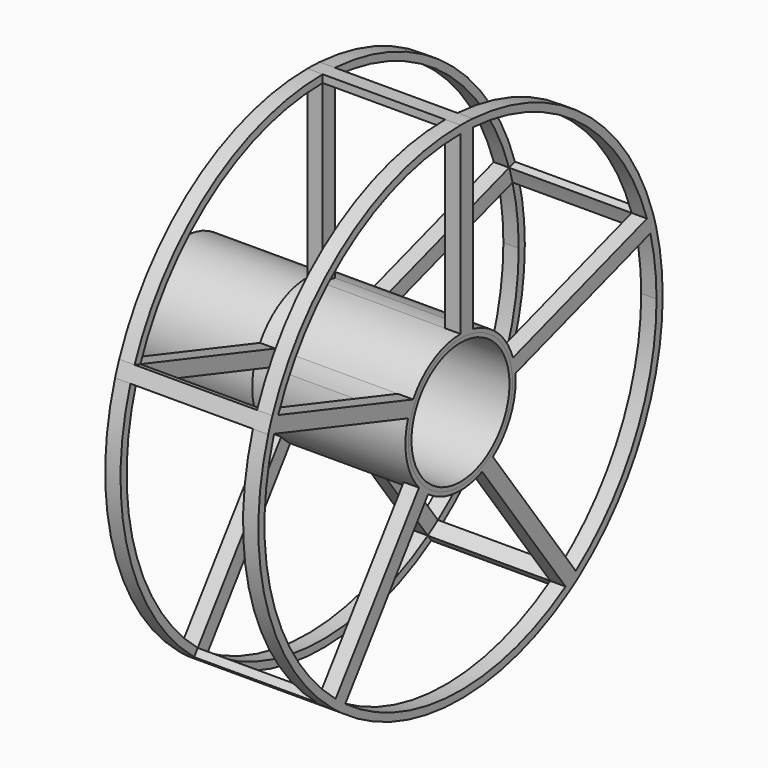
from build123d import *

# Parameters (mm, degrees)
F0_R          = 13.49375
F1_DEPTH      = 3.175
F2_DEPTH      = 28.575
F3_START      = 28.575
F3_DEPTH      = 3.175
F0_R_2        = 12.7
F4_DEPTH      = 31.75
F4_DEPTH_BACK = 25.4
F5_DEPTH      = 31.75


with BuildPart() as f1:
    # F0 (on Right) → F1 (new body)
    with BuildSketch(Plane.YZ):
        with BuildLine():
            ThreePointArc((3.175, 50.700684), (31.129836, 40.144406), (48.313671, 15.698063))
            Line((48.313671, 15.698063), (49.823473, 16.188628))
            ThreePointArc((49.823473, 16.188628), (32.063351, 41.429358), (3.175, 52.291199))
            Line((3.175, 52.291199), (3.175, 50.700684))
        make_face()
        with BuildLine():
            Line((28.167367, -44.170687), (27.232485, -42.883933))
            ThreePointArc((27.232485, -42.883933), (-1.588276, -50.775165), (-29.859491, -41.098063))
            Line((-29.859491, -41.098063), (-30.7926, -42.382378))
            ThreePointArc((-30.7926, -42.382378), (-1.58823, -52.363419), (28.167367, -44.170687))
        make_face()
        with BuildLine():
            ThreePointArc((0, 50.8), (1.588276, 50.775165), (3.175, 50.700684))
            Line((3.175, 50.700684), (3.175, 52.291199))
            ThreePointArc((3.175, 52.291199), (1.58823, 52.363419), (0, 52.3875))
            Line((0, 52.3875), (0, 50.8))
        make_face()
        with BuildLine():
            ThreePointArc((48.313671, 15.698063), (48.780856, 14.179848), (49.200345, 12.647769))
            Line((49.200345, 12.647769), (50.713015, 13.139265))
            ThreePointArc((50.713015, 13.139265), (50.291361, 14.67069), (49.823473, 16.188628))
            Line((49.823473, 16.188628), (48.313671, 15.698063))
        make_face()
        with BuildLine():
            ThreePointArc((49.200345, 12.647769), (50.3985, 6.374264), (50.8, 0))
            ThreePointArc((50.8, 0), (45.263131, -23.062717), (29.859491, -41.098063))
            Line((29.859491, -41.098063), (30.7926, -42.382378))
            ThreePointArc((30.7926, -42.382378), (46.677604, -23.783427), (52.3875, 0))
            ThreePointArc((52.3875, 0), (51.967193, 6.622767), (50.713015, 13.139265))
            Line((50.713015, 13.139265), (49.200345, 12.647769))
        make_face()
        with BuildLine():
            ThreePointArc((-47.238087, 18.686977), (-28.55995, 42.011537), (0, 50.8))
            Line((0, 50.8), (0, 52.3875))
            ThreePointArc((0, 52.3875), (-29.493541, 43.296434), (-48.750757, 19.178474))
            Line((-48.750757, 19.178474), (-47.238087, 18.686977))
        make_face()
        with BuildLine():
            Line((-33.304625, -40.438251), (-32.369743, -39.151497))
            ThreePointArc((-32.369743, -39.151497), (-48.780856, -14.179848), (-48.313671, 15.698063))
            Line((-48.313671, 15.698063), (-49.823473, 16.188628))
            ThreePointArc((-49.823473, 16.188628), (-50.291361, -14.67069), (-33.304625, -40.438251))
        make_face()
        with BuildLine():
            ThreePointArc((-48.313671, 15.698063), (-47.799247, 17.20093), (-47.238087, 18.686977))
            Line((-47.238087, 18.686977), (-48.750757, 19.178474))
            ThreePointArc((-48.750757, 19.178474), (-49.309781, 17.691683), (-49.823473, 16.188628))
            Line((-49.823473, 16.188628), (-48.313671, 15.698063))
        make_face()
        with BuildLine():
            Line((30.7926, -42.382378), (29.859491, -41.098063))
            ThreePointArc((29.859491, -41.098063), (28.55995, -42.011537), (27.232485, -42.883933))
            Line((27.232485, -42.883933), (28.167367, -44.170687))
            ThreePointArc((28.167367, -44.170687), (29.493541, -43.296434), (30.7926, -42.382378))
        make_face()
        with BuildLine():
            ThreePointArc((-32.369743, -39.151497), (-31.129836, -40.144406), (-29.859491, -41.098063))
            Line((-29.859491, -41.098063), (-8.397982, -11.55883))
            ThreePointArc((-8.397982, -11.55883), (-9.63774, -10.547352), (-10.756628, -9.403596))
            Line((-10.756628, -9.403596), (-32.369743, -39.151497))
        make_face()
        with BuildLine():
            Line((14.22959, 1.285081), (49.200345, 12.647769))
            ThreePointArc((49.200345, 12.647769), (48.780856, 14.179848), (48.313671, 15.698063))
            Line((48.313671, 15.698063), (13.58822, 4.41508))
            ThreePointArc((13.58822, 4.41508), (13.996673, 2.868065), (14.22959, 1.285081))
        make_face()
        with BuildLine():
            ThreePointArc((27.232485, -42.883933), (28.55995, -42.011537), (29.859491, -41.098063))
            Line((29.859491, -41.098063), (8.397982, -11.55883))
            ThreePointArc((8.397982, -11.55883), (7.052902, -12.425346), (5.61937, -13.136032))
            Line((5.61937, -13.136032), (27.232485, -42.883933))
        make_face()
        with BuildLine():
            Line((3.175, 13.930256), (3.175, 50.700684))
            ThreePointArc((3.175, 50.700684), (1.588276, 50.775165), (0, 50.8))
            Line((0, 50.8), (0, 14.2875))
            ThreePointArc((0, 14.2875), (1.597517, 14.197908), (3.175, 13.930256))
        make_face()
        with BuildLine():
            Line((-30.7926, -42.382378), (-29.859491, -41.098063))
            ThreePointArc((-29.859491, -41.098063), (-31.129836, -40.144406), (-32.369743, -39.151497))
            Line((-32.369743, -39.151497), (-33.304625, -40.438251))
            ThreePointArc((-33.304625, -40.438251), (-32.063351, -41.429358), (-30.7926, -42.382378))
        make_face()
        with BuildLine():
            ThreePointArc((14.2875, 0), (14.273015, 0.643193), (14.22959, 1.285081))
            ThreePointArc((14.22959, 1.285081), (13.996673, 2.868065), (13.58822, 4.41508))
            ThreePointArc((13.58822, 4.41508), (9.63774, 10.547352), (3.175, 13.930256))
            ThreePointArc((3.175, 13.930256), (1.597517, 14.197908), (0, 14.2875))
            ThreePointArc((0, 14.2875), (-7.052902, 12.425346), (-12.267332, 7.32429))
            ThreePointArc((-12.267332, 7.32429), (-13.009353, 5.906724), (-13.58822, 4.41508))
            ThreePointArc((-13.58822, 4.41508), (-13.996673, -2.868065), (-10.756628, -9.403596))
            ThreePointArc((-10.756628, -9.403596), (-9.63774, -10.547352), (-8.397982, -11.55883))
            ThreePointArc((-8.397982, -11.55883), (-1.597517, -14.197908), (5.61937, -13.136032))
            ThreePointArc((5.61937, -13.136032), (7.052902, -12.425346), (8.397982, -11.55883))
            ThreePointArc((8.397982, -11.55883), (12.730256, -6.486389), (14.2875, 0))
        make_face()
        Circle(F0_R, mode=Mode.SUBTRACT)
        with BuildLine():
            Line((-12.267332, 7.32429), (-47.238087, 18.686977))
            ThreePointArc((-47.238087, 18.686977), (-47.799247, 17.20093), (-48.313671, 15.698063))
            Line((-48.313671, 15.698063), (-13.58822, 4.41508))
            ThreePointArc((-13.58822, 4.41508), (-13.009353, 5.906724), (-12.267332, 7.32429))
        make_face()
    extrude(amount=F1_DEPTH)

    # F0 (on Right) → F2 (join)
    with BuildSketch(Plane.YZ):
        with BuildLine():
            ThreePointArc((48.313671, 15.698063), (48.780856, 14.179848), (49.200345, 12.647769))
            Line((49.200345, 12.647769), (50.713015, 13.139265))
            ThreePointArc((50.713015, 13.139265), (50.291361, 14.67069), (49.823473, 16.188628))
            Line((49.823473, 16.188628), (48.313671, 15.698063))
        make_face()
        with BuildLine():
            Line((-30.7926, -42.382378), (-29.859491, -41.098063))
            ThreePointArc((-29.859491, -41.098063), (-31.129836, -40.144406), (-32.369743, -39.151497))
            Line((-32.369743, -39.151497), (-33.304625, -40.438251))
            ThreePointArc((-33.304625, -40.438251), (-32.063351, -41.429358), (-30.7926, -42.382378))
        make_face()
        with BuildLine():
            ThreePointArc((0, 50.8), (1.588276, 50.775165), (3.175, 50.700684))
            Line((3.175, 50.700684), (3.175, 52.291199))
            ThreePointArc((3.175, 52.291199), (1.58823, 52.363419), (0, 52.3875))
            Line((0, 52.3875), (0, 50.8))
        make_face()
        with BuildLine():
            Line((30.7926, -42.382378), (29.859491, -41.098063))
            ThreePointArc((29.859491, -41.098063), (28.55995, -42.011537), (27.232485, -42.883933))
            Line((27.232485, -42.883933), (28.167367, -44.170687))
            ThreePointArc((28.167367, -44.170687), (29.493541, -43.296434), (30.7926, -42.382378))
        make_face()
        with BuildLine():
            ThreePointArc((-48.313671, 15.698063), (-47.799247, 17.20093), (-47.238087, 18.686977))
            Line((-47.238087, 18.686977), (-48.750757, 19.178474))
            ThreePointArc((-48.750757, 19.178474), (-49.309781, 17.691683), (-49.823473, 16.188628))
            Line((-49.823473, 16.188628), (-48.313671, 15.698063))
        make_face()
        with BuildLine():
            ThreePointArc((14.2875, 0), (14.273015, 0.643193), (14.22959, 1.285081))
            ThreePointArc((14.22959, 1.285081), (13.996673, 2.868065), (13.58822, 4.41508))
            ThreePointArc((13.58822, 4.41508), (9.63774, 10.547352), (3.175, 13.930256))
            ThreePointArc((3.175, 13.930256), (1.597517, 14.197908), (0, 14.2875))
            ThreePointArc((0, 14.2875), (-7.052902, 12.425346), (-12.267332, 7.32429))
            ThreePointArc((-12.267332, 7.32429), (-13.009353, 5.906724), (-13.58822, 4.41508))
            ThreePointArc((-13.58822, 4.41508), (-13.996673, -2.868065), (-10.756628, -9.403596))
            ThreePointArc((-10.756628, -9.403596), (-9.63774, -10.547352), (-8.397982, -11.55883))
            ThreePointArc((-8.397982, -11.55883), (-1.597517, -14.197908), (5.61937, -13.136032))
            ThreePointArc((5.61937, -13.136032), (7.052902, -12.425346), (8.397982, -11.55883))
            ThreePointArc((8.397982, -11.55883), (12.730256, -6.486389), (14.2875, 0))
        make_face()
        Circle(F0_R, mode=Mode.SUBTRACT)
    extrude(amount=F2_DEPTH)

    # F0 (on Right) → F3 (join)
    with BuildSketch(Plane.YZ.offset(F3_START)):
        with BuildLine():
            ThreePointArc((14.2875, 0), (14.273015, 0.643193), (14.22959, 1.285081))
            ThreePointArc((14.22959, 1.285081), (13.996673, 2.868065), (13.58822, 4.41508))
            ThreePointArc((13.58822, 4.41508), (9.63774, 10.547352), (3.175, 13.930256))
            ThreePointArc((3.175, 13.930256), (1.597517, 14.197908), (0, 14.2875))
            ThreePointArc((0, 14.2875), (-7.052902, 12.425346), (-12.267332, 7.32429))
            ThreePointArc((-12.267332, 7.32429), (-13.009353, 5.906724), (-13.58822, 4.41508))
            ThreePointArc((-13.58822, 4.41508), (-13.996673, -2.868065), (-10.756628, -9.403596))
            ThreePointArc((-10.756628, -9.403596), (-9.63774, -10.547352), (-8.397982, -11.55883))
            ThreePointArc((-8.397982, -11.55883), (-1.597517, -14.197908), (5.61937, -13.136032))
            ThreePointArc((5.61937, -13.136032), (7.052902, -12.425346), (8.397982, -11.55883))
            ThreePointArc((8.397982, -11.55883), (12.730256, -6.486389), (14.2875, 0))
        make_face()
        Circle(F0_R, mode=Mode.SUBTRACT)
        with BuildLine():
            Line((-12.267332, 7.32429), (-47.238087, 18.686977))
            ThreePointArc((-47.238087, 18.686977), (-47.799247, 17.20093), (-48.313671, 15.698063))
            Line((-48.313671, 15.698063), (-13.58822, 4.41508))
            ThreePointArc((-13.58822, 4.41508), (-13.009353, 5.906724), (-12.267332, 7.32429))
        make_face()
        with BuildLine():
            ThreePointArc((-47.238087, 18.686977), (-28.55995, 42.011537), (0, 50.8))
            Line((0, 50.8), (0, 52.3875))
            ThreePointArc((0, 52.3875), (-29.493541, 43.296434), (-48.750757, 19.178474))
            Line((-48.750757, 19.178474), (-47.238087, 18.686977))
        make_face()
        with BuildLine():
            Line((-30.7926, -42.382378), (-29.859491, -41.098063))
            ThreePointArc((-29.859491, -41.098063), (-31.129836, -40.144406), (-32.369743, -39.151497))
            Line((-32.369743, -39.151497), (-33.304625, -40.438251))
            ThreePointArc((-33.304625, -40.438251), (-32.063351, -41.429358), (-30.7926, -42.382378))
        make_face()
        with BuildLine():
            ThreePointArc((-48.313671, 15.698063), (-47.799247, 17.20093), (-47.238087, 18.686977))
            Line((-47.238087, 18.686977), (-48.750757, 19.178474))
            ThreePointArc((-48.750757, 19.178474), (-49.309781, 17.691683), (-49.823473, 16.188628))
            Line((-49.823473, 16.188628), (-48.313671, 15.698063))
        make_face()
        with BuildLine():
            Line((28.167367, -44.170687), (27.232485, -42.883933))
            ThreePointArc((27.232485, -42.883933), (-1.588276, -50.775165), (-29.859491, -41.098063))
            Line((-29.859491, -41.098063), (-30.7926, -42.382378))
            ThreePointArc((-30.7926, -42.382378), (-1.58823, -52.363419), (28.167367, -44.170687))
        make_face()
        with BuildLine():
            ThreePointArc((27.232485, -42.883933), (28.55995, -42.011537), (29.859491, -41.098063))
            Line((29.859491, -41.098063), (8.397982, -11.55883))
            ThreePointArc((8.397982, -11.55883), (7.052902, -12.425346), (5.61937, -13.136032))
            Line((5.61937, -13.136032), (27.232485, -42.883933))
        make_face()
        with BuildLine():
            Line((30.7926, -42.382378), (29.859491, -41.098063))
            ThreePointArc((29.859491, -41.098063), (28.55995, -42.011537), (27.232485, -42.883933))
            Line((27.232485, -42.883933), (28.167367, -44.170687))
            ThreePointArc((28.167367, -44.170687), (29.493541, -43.296434), (30.7926, -42.382378))
        make_face()
        with BuildLine():
            ThreePointArc((3.175, 50.700684), (31.129836, 40.144406), (48.313671, 15.698063))
            Line((48.313671, 15.698063), (49.823473, 16.188628))
            ThreePointArc((49.823473, 16.188628), (32.063351, 41.429358), (3.175, 52.291199))
            Line((3.175, 52.291199), (3.175, 50.700684))
        make_face()
        with BuildLine():
            Line((3.175, 13.930256), (3.175, 50.700684))
            ThreePointArc((3.175, 50.700684), (1.588276, 50.775165), (0, 50.8))
            Line((0, 50.8), (0, 14.2875))
            ThreePointArc((0, 14.2875), (1.597517, 14.197908), (3.175, 13.930256))
        make_face()
        with BuildLine():
            ThreePointArc((0, 50.8), (1.588276, 50.775165), (3.175, 50.700684))
            Line((3.175, 50.700684), (3.175, 52.291199))
            ThreePointArc((3.175, 52.291199), (1.58823, 52.363419), (0, 52.3875))
            Line((0, 52.3875), (0, 50.8))
        make_face()
        with BuildLine():
            Line((14.22959, 1.285081), (49.200345, 12.647769))
            ThreePointArc((49.200345, 12.647769), (48.780856, 14.179848), (48.313671, 15.698063))
            Line((48.313671, 15.698063), (13.58822, 4.41508))
            ThreePointArc((13.58822, 4.41508), (13.996673, 2.868065), (14.22959, 1.285081))
        make_face()
        with BuildLine():
            Line((-33.304625, -40.438251), (-32.369743, -39.151497))
            ThreePointArc((-32.369743, -39.151497), (-48.780856, -14.179848), (-48.313671, 15.698063))
            Line((-48.313671, 15.698063), (-49.823473, 16.188628))
            ThreePointArc((-49.823473, 16.188628), (-50.291361, -14.67069), (-33.304625, -40.438251))
        make_face()
        with BuildLine():
            ThreePointArc((-32.369743, -39.151497), (-31.129836, -40.144406), (-29.859491, -41.098063))
            Line((-29.859491, -41.098063), (-8.397982, -11.55883))
            ThreePointArc((-8.397982, -11.55883), (-9.63774, -10.547352), (-10.756628, -9.403596))
            Line((-10.756628, -9.403596), (-32.369743, -39.151497))
        make_face()
        with BuildLine():
            ThreePointArc((48.313671, 15.698063), (48.780856, 14.179848), (49.200345, 12.647769))
            Line((49.200345, 12.647769), (50.713015, 13.139265))
            ThreePointArc((50.713015, 13.139265), (50.291361, 14.67069), (49.823473, 16.188628))
            Line((49.823473, 16.188628), (48.313671, 15.698063))
        make_face()
        with BuildLine():
            ThreePointArc((49.200345, 12.647769), (50.3985, 6.374264), (50.8, 0))
            ThreePointArc((50.8, 0), (45.263131, -23.062717), (29.859491, -41.098063))
            Line((29.859491, -41.098063), (30.7926, -42.382378))
            ThreePointArc((30.7926, -42.382378), (46.677604, -23.783427), (52.3875, 0))
            ThreePointArc((52.3875, 0), (51.967193, 6.622767), (50.713015, 13.139265))
            Line((50.713015, 13.139265), (49.200345, 12.647769))
        make_face()
    extrude(amount=F3_DEPTH)


with BuildPart() as f4:
    # F0 (on Right) → F4 (new body, two sides)
    with BuildSketch(Plane.YZ) as f4_sk:
        Circle(F0_R)
        Circle(F0_R_2, mode=Mode.SUBTRACT)
    extrude(amount=F4_DEPTH)
    extrude(f4_sk.sketch, amount=-F4_DEPTH_BACK)


with BuildPart() as f5:
    # F0 (on Right) → F5 (new body)
    with BuildSketch(Plane.YZ):
        Circle(F0_R)
        Circle(F0_R_2, mode=Mode.SUBTRACT)
    extrude(amount=F5_DEPTH)


solid = Compound([f1.part, f4.part, f5.part])
